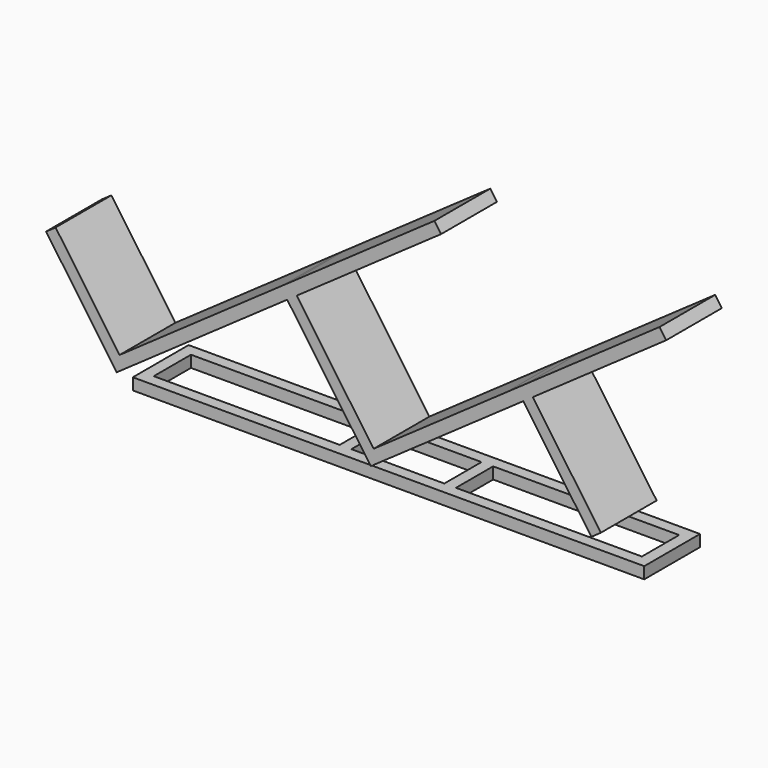
from build123d import *

# Parameters (mm, degrees)
F1_DEPTH = 15
F0_W     = 2.5
F0_H     = 2.5
F2_W     = 20
F2_H     = 10
F2_W_2   = 40
F3_DEPTH = 70


# Not quite as in the source:
# - a feature of the source that left no trace in its solid (it failed there, or was rolled back) is left out


with BuildPart() as f1:
    # F0 (on Front) → F1 (new body)
    with BuildSketch(Plane.XZ):
        Polygon((-28.0954666037, 23.5771734984), (-21.7977855629, 27.9868572364), (-19.7499054522, 29.4207983273), (-21.1838465431, 31.468678438), (-22.9467930342, 30.2342500155), (-57.8463816277, 5.7972950019), (-71.6116508746, 25.456136839), (-73.6595309853, 24.0221957481), (-58.4603206476, 2.3154738003), align=None)
        Polygon((-21.1838465431, 31.468678438), (-19.7499054522, 29.4207983273), (11.3069104876, 51.1670149611), (9.8729693967, 53.2148950719), align=None)
        Polygon((-21.7977855629, 27.9868572364), (-3.9516960007, 2.5), (-3.5589586403, 2.5), (23.6399283018, 21.5448656678), (28.9750478761, 25.280556611), (31.0229279868, 26.7144977018), (29.588986896, 28.7623778126), (25.1048015935, 25.6225174611), (-3.2085503448, 5.7972950019), (-19.7499054522, 29.4207983273), align=None)
        Polygon((31.0229279868, 26.7144977018), (28.9750478761, 25.280556611), (43.6214308849, 4.363353911), (45.6693109956, 5.7972950019), align=None)
        Polygon((29.588986896, 28.7623778126), (31.0229279868, 26.7144977018), (59.7092352027, 46.8008662578), (58.2752941118, 48.8487463685), align=None)
    extrude(amount=F1_DEPTH)


with BuildPart() as f1b:
    # F0 (on Front) → F1, piece 2 (new body)
    with BuildSketch(Plane.XZ):
        Polygon((-52.5, 2.5), (-52.5, 0), (52.5, 0), (52.5, 2.5), (-3.5589586403, 2.5), (-3.8224893646, 2.3154738003), (-3.9516960007, 2.5), align=None)
        with Locations((53.75, 1.25)):
            Rectangle(F0_W, F0_H)
        with Locations((-53.75, 1.25)):
            Rectangle(F0_W, F0_H)
    extrude(amount=F1_DEPTH)

    # F2 (on Top) → F3 (cut)
    with BuildSketch(Plane.XY):
        with Locations((0, -7.5)):
            Rectangle(F2_W, F2_H)
        with Locations((32.5, -7.5)):
            Rectangle(F2_W_2, F2_H)
        with Locations((-32.5, -7.5)):
            Rectangle(F2_W_2, F2_H)
    extrude(amount=F3_DEPTH, mode=Mode.SUBTRACT)


solid = Compound([f1.part, f1b.part])
